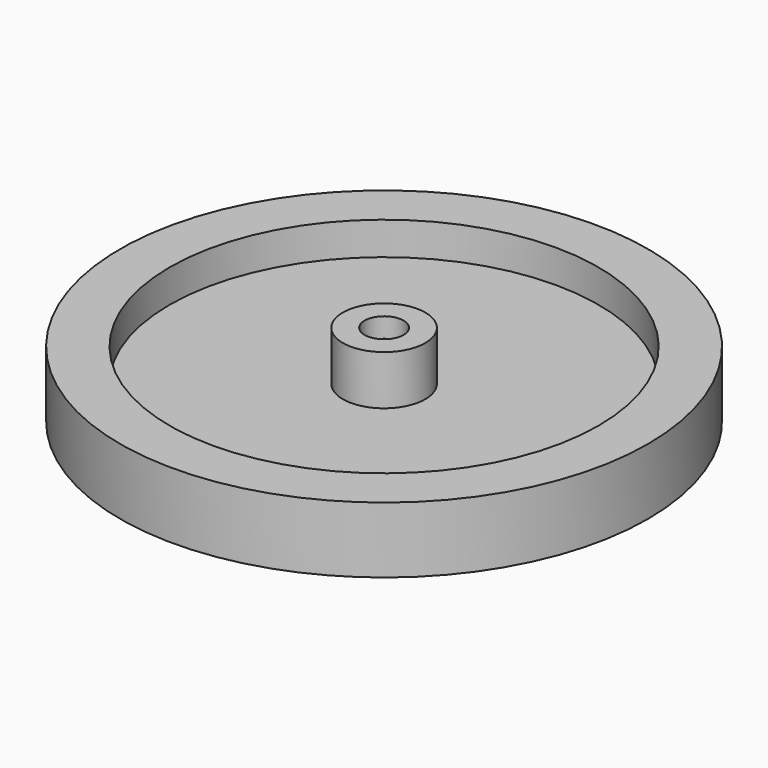
from build123d import *
from build123d import SkipClean  # not in build123d's __all__

# Parameters (mm, degrees)
F0_R          = 40.64
F1_DEPTH      = 10.16
F2_R          = 33.02
F3_DEPTH      = 5.08
F5_DEPTH      = 10.16
F6_R          = 6.35
F6_R_2        = 2.9972
F7_DEPTH      = 7.62
F7_DEPTH_BACK = 0.0127
F8_W          = 7.62
F8_H          = 2.54
F9_DEPTH      = 9.652


# Not quite as in the source:
# - after a boolean that leaves OpenCascade's solid faulty, fix() repairs it


with BuildPart() as f1:
    # F0 (on Top) → F1 (new body)
    with BuildSketch(Plane.XY):
        Circle(F0_R)
    extrude(amount=F1_DEPTH)

    # F2 (on face) → F3 (cut)
    with BuildSketch(Plane.XY.offset(10.16)):
        Circle(F2_R)
    extrude(amount=-F3_DEPTH, mode=Mode.SUBTRACT)

    # F4 (on face) → F5 (cut)
    with BuildSketch(Plane(origin=(0, 0, 0), x_dir=(1, 0, 0), z_dir=(0, 0, -1))):
        with BuildLine():
            Line((2.3139107243, -1.905), (-2.3139107243, -1.905))
            ThreePointArc((-2.3139107243, -1.905), (0, -2.9972), (2.3139107243, -1.905))
        make_face()
        with BuildLine():
            ThreePointArc((2.3139107243, -1.905), (2.8212108272, -1.0119176392), (2.9972, 0))
            ThreePointArc((2.9972, 0), (-1.0119176392, 2.8212108272), (-2.3139107243, -1.905))
            Line((-2.3139107243, -1.905), (2.3139107243, -1.905))
        make_face()
    extrude(amount=-F5_DEPTH, mode=Mode.SUBTRACT)

    # F6 (on face) → F7 (join, two sides)
    with BuildSketch(Plane.XY.offset(5.08)) as f7_sk:
        Circle(F6_R)
        Circle(F6_R_2, mode=Mode.SUBTRACT)
    with SkipClean():  # cleaning this boolean's faces spoils the solid; the shape is the same uncleaned
        extrude(amount=F7_DEPTH)
        extrude(f7_sk.sketch, amount=-F7_DEPTH_BACK)

    # F8 (on Top) → F9 (join)
    with BuildSketch(Plane.XY):
        with Locations((0, 3.175)):
            Rectangle(F8_W, F8_H)
    extrude(amount=F9_DEPTH)

    add(f1.part.fix(), mode=Mode.REPLACE)


solid = f1.part
